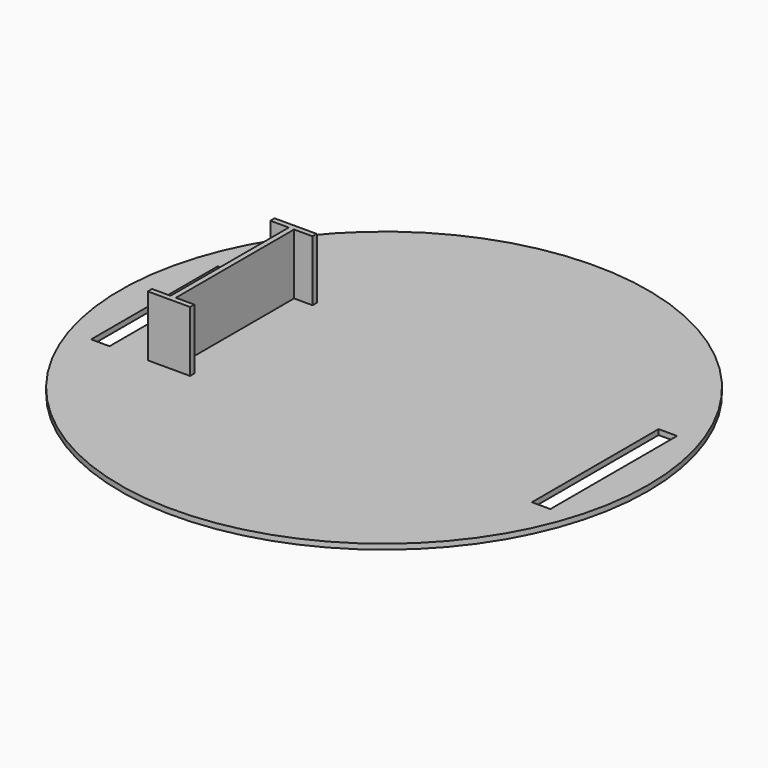
from build123d import *

# Parameters (mm, degrees)
F0_R     = 100
F0_W     = 7
F0_H     = 60
F0_H_2   = 2
F0_W_2   = 2
F0_H_3   = 56
F1_DEPTH = 2
F2_DEPTH = 25


# Not quite as in the source:
# - a feature names something its author has since deleted; it is built from what else it names


with BuildPart() as f1:
    # F0 (on Top) → F1 (new body)
    with BuildSketch(Plane.XY):
        Circle(F0_R)
        with Locations((-83.5, 0)):
            Rectangle(F0_W, F0_H, mode=Mode.SUBTRACT)
        Polygon((-58.5, 30), (-56.5, 30), (-49.5, 30), (-49.5, 28), (-56.5, 28), (-56.5, -28), (-49.5, -28), (-49.5, -30), (-56.5, -30), (-58.5, -30), (-65.5, -30), (-65.5, -28), (-58.5, -28), (-58.5, 28), (-65.5, 28), (-65.5, 30), align=None, mode=Mode.SUBTRACT)
        with Locations((83.5, 0)):
            Rectangle(F0_W, F0_H, mode=Mode.SUBTRACT)
        with Locations((-62, -29)):
            Rectangle(F0_W, F0_H_2)
        with Locations((-57.5, -29)):
            Rectangle(F0_W_2, F0_H_2)
        with Locations((-53, -29)):
            Rectangle(F0_W, F0_H_2)
        with Locations((-57.5, 0)):
            Rectangle(F0_W_2, F0_H_3)
        with Locations((-62, 29)):
            Rectangle(F0_W, F0_H_2)
        with Locations((-57.5, 29)):
            Rectangle(F0_W_2, F0_H_2)
        with Locations((-53, 29)):
            Rectangle(F0_W, F0_H_2)
    extrude(amount=F1_DEPTH)

    # F0 (on Top) → F2 (join)
    with BuildSketch(Plane.XY):
        with Locations((-62, 29)):
            Rectangle(F0_W, F0_H_2)
        with Locations((-57.5, 29)):
            Rectangle(F0_W_2, F0_H_2)
        with Locations((-53, 29)):
            Rectangle(F0_W, F0_H_2)
        with Locations((-57.5, 0)):
            Rectangle(F0_W_2, F0_H_3)
        with Locations((-62, -29)):
            Rectangle(F0_W, F0_H_2)
        with Locations((-57.5, -29)):
            Rectangle(F0_W_2, F0_H_2)
        with Locations((-53, -29)):
            Rectangle(F0_W, F0_H_2)
    extrude(amount=F2_DEPTH)


solid = f1.part
